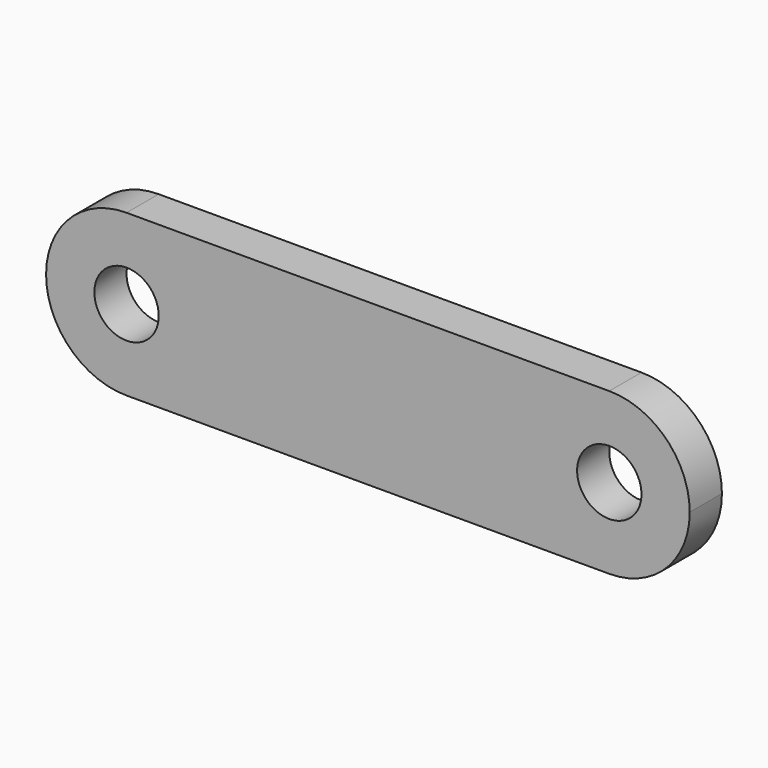
from build123d import *

# Parameters (mm, degrees)
F0_W     = 80
F0_H     = 20
F1_DEPTH = 5
F2_R     = 9.99999
F3_R     = 4
F4_DEPTH = 5.001


# Not quite as in the source:
# - a fillet or chamfer is up to 0.001 mm smaller than in the source, because OpenCascade refuses the exact size


with BuildPart() as f1:
    # F0 (on Front) → F1 (new body)
    with BuildSketch(Plane.XZ):
        with Locations((40, 10)):
            Rectangle(F0_W, F0_H)
    extrude(amount=F1_DEPTH)

    # F2 (radius 10 in the source; OpenCascade refuses exactly that, so slightly less here)
    f2_edges = [f1.edges().sort_by_distance(p)[0] for p in [
        (80, -2.5, 20),
        (80, -2.5, 0),
        (0, -2.5, 20),
        (0, -2.5, 0),
    ]]
    fillet(f2_edges, radius=F2_R)

    # F3 (on face) → F4 (cut, through all)
    with BuildSketch(Plane.XZ.offset(5)):
        with Locations((10, 10)):
            Circle(F3_R)
        with Locations((70, 10)):
            Circle(F3_R)
    extrude(amount=-F4_DEPTH, mode=Mode.SUBTRACT)


solid = f1.part
